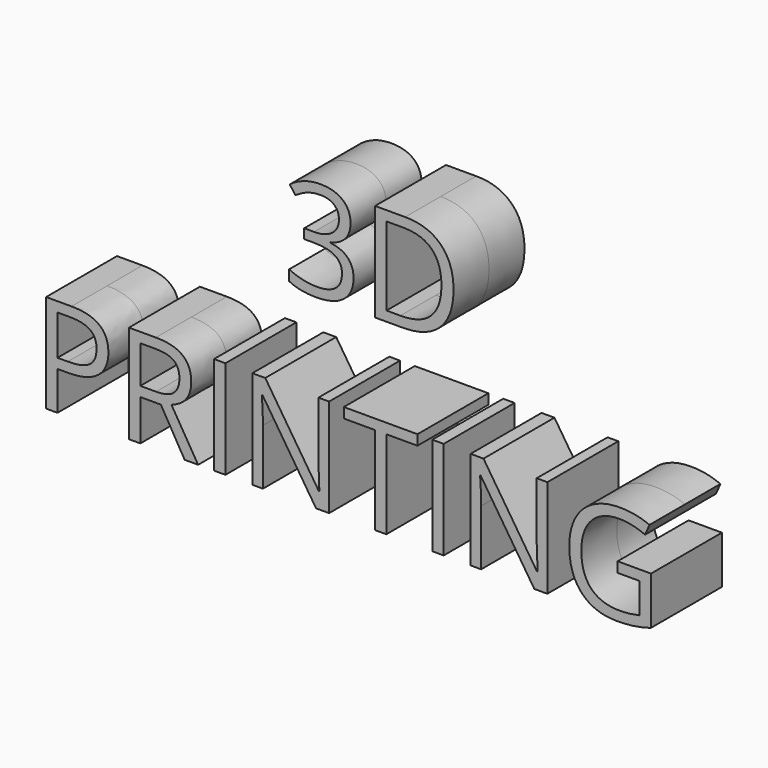
from build123d import *

# Parameters (mm, degrees)
F0_TEXT_SIZE = 39.4222378317
F1_DEPTH     = 12.7


# Not quite as in the source:
# - Text() gives the source's letters only with a copy of the font that has no kerning and outlines rounded to 1/6400 em; it was checked with that copy


with BuildPart() as f1:
    # F0 (on Front) → F1 (new body, symmetric)
    with BuildSketch(Plane.XZ):
        with Locations((48.1768151876, 0)):
            Text('3D', F0_TEXT_SIZE, font='Open Sans', text_align=(TextAlign.LEFT, TextAlign.BOTTOM))
        with Locations((-23.5285395934, -53.6142434511)):
            Text('PRINTING', F0_TEXT_SIZE, font='Open Sans', text_align=(TextAlign.LEFT, TextAlign.BOTTOM))
    extrude(amount=F1_DEPTH, both=True)


solid = f1.part
